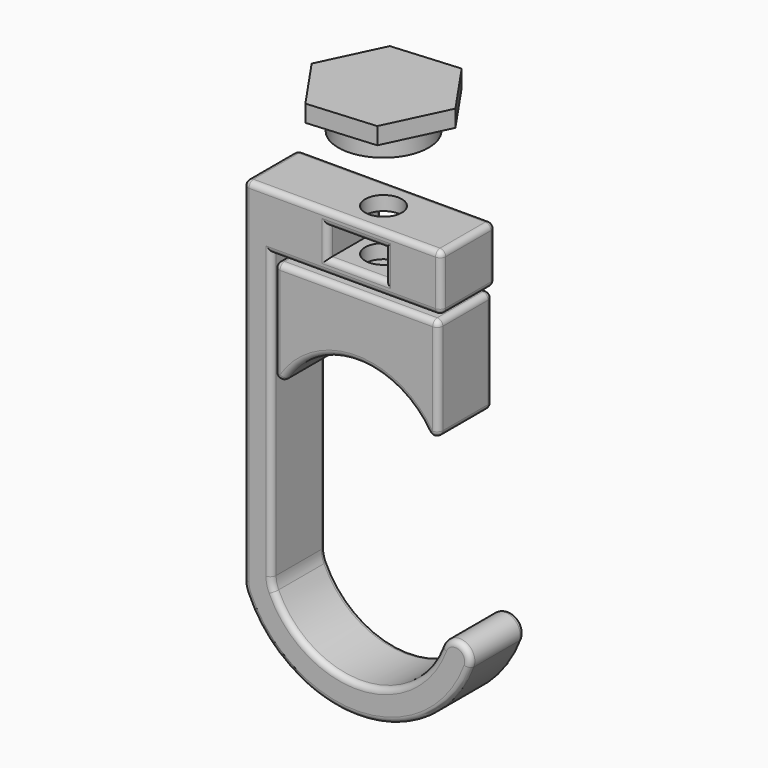
from build123d import *

# Parameters (mm, degrees)
F1_DEPTH  = 6
F3_R      = 3.25
F4_DEPTH  = 15.8
F5_W      = 10.1
F5_H      = 5
F6_DEPTH  = 25
F8_DEPTH  = 5
F10_DEPTH = 12
F12_R     = 1
F12_2_R   = 1


with BuildPart() as f1:
    # F0 (on Front) → F1 (new body, symmetric)
    with BuildSketch(Plane.XZ):
        with BuildLine():
            Line((-15, 0.9851886679), (-15, 51.4083372368))
            Line((-15, 51.4083372368), (15, 51.4083372368))
            Line((15, 51.4083372368), (15, 61.4083372368))
            Line((15, 61.4083372368), (-20, 61.4083372368))
            Line((-20, 61.4083372368), (-20, -0.8958087804))
            ThreePointArc((-20, -0.8958087804), (-19.8968961431, -1.9059613249), (-19.5918367347, -2.8744536202))
            ThreePointArc((-19.5918367347, -2.8744536202), (0.5486358136, -15.7585130867), (20, -1.8559214543))
            ThreePointArc((20, -1.8559214543), (18.4279607271, 1.5720392729), (15, 0))
            ThreePointArc((15, 0), (0.5940911198, -10.4212023249), (-14.5454545455, -1.0978002844))
            ThreePointArc((-14.5454545455, -1.0978002844), (-14.8850421046, -0.0808149139), (-15, 0.9851886679))
        make_face()
    extrude(amount=F1_DEPTH, both=True)


with BuildPart() as f1b:
    # F0 (on Front) → F1, piece 2 (new body, symmetric)
    with BuildSketch(Plane.XZ):
        with BuildLine():
            Line((14.5, 50.4083372368), (-14.5, 50.4083372368))
            Line((-14.5, 50.4083372368), (-14.5, 28.4083372368))
            ThreePointArc((-14.5, 28.4083372368), (0, 39.5677643628), (14.5, 28.4083372368))
            Line((14.5, 28.4083372368), (14.5, 50.4083372368))
        make_face()
    extrude(amount=F1_DEPTH, both=True)


with BuildPart() as f2:
    # F0 (on Front) → F2 (revolve)
    with BuildSketch(Plane.XZ):
        Polygon((12, 80.0677643628), (0, 80.0677643628), (0, 73.0677643628), (8, 73.0677643628), (8, 77.0677643628), (12, 77.0677643628), align=None)
    revolve(axis=Axis((0, 0, 76.5677643628), (0, 0, -1)))

    # F7 (on face) → F8 (cut)
    with BuildSketch(Plane(origin=(0, 0, 73.0677643628), x_dir=(1, 0, 0), z_dir=(0, 0, -1))):
        Polygon((5.05, -2.9156188594), (5.05, 2.9156188594), (0, 5.8312377188), (-5.05, 2.9156188594), (-5.05, -2.9156188594), (0, -5.8312377188), align=None)
    extrude(amount=-F8_DEPTH, mode=Mode.SUBTRACT)


with BuildPart() as f4_tool:
    # F3 (on face) → F4 (new body)
    with BuildSketch(Plane.XY.offset(61.4083372368)):
        Circle(F3_R)
    extrude(amount=-F4_DEPTH)


with BuildPart() as f1_1:
    add(f1.part)

    # F4: cut by f4_tool
    add(f4_tool.part, mode=Mode.SUBTRACT)

    # F5 (on face) → F6 (cut)
    with BuildSketch(Plane.XZ.offset(6)):
        with Locations((0, 56.4083372368)):
            Rectangle(F5_W, F5_H)
    extrude(amount=-F6_DEPTH, mode=Mode.SUBTRACT)

    # F12
    f12_edges = [f1_1.edges().sort_by_distance(p)[0] for p in [
        (-14.885042, -6, -0.080815),
        (0.594091, -6, -10.421202),
        (-15, -6, 26.196763),
        (18.427961, -6, 1.572039),
        (0, -6, 51.408337),
        (0.548636, -6, -15.758513),
        (15, -6, 56.408337),
        (-19.896896, -6, -1.905961),
        (-2.5, -6, 61.408337),
        (-20, -6, 30.256264),
        (0, -6, 58.908337),
        (-5.05, -6, 56.408337),
        (0, -6, 53.908337),
        (5.05, -6, 56.408337),
        (-14.885042, 6, -0.080815),
        (0.594091, 6, -10.421202),
        (-15, 6, 26.196763),
        (18.427961, 6, 1.572039),
        (0, 6, 51.408337),
        (0.548636, 6, -15.758513),
        (15, 6, 56.408337),
        (-19.896896, 6, -1.905961),
        (-2.5, 6, 61.408337),
        (-20, 6, 30.256264),
        (0, 6, 58.908337),
        (-5.05, 6, 56.408337),
        (0, 6, 53.908337),
        (5.05, 6, 56.408337),
        (15, 0, 51.408337),
        (15, 0, 61.408337),
        (-20, 0, 61.408337),
        (-20, 0, -0.895809),
    ]]
    fillet(f12_edges, radius=F12_R)


with BuildPart() as f1b_1:
    add(f1b.part)

    # F4: cut by f4_tool
    add(f4_tool.part, mode=Mode.SUBTRACT)

    # F12#2
    f12_2_edges = [f1b_1.edges().sort_by_distance(p)[0] for p in [
        (14.5, -6, 39.408337),
        (0, -6, 50.408337),
        (-14.5, -6, 39.408337),
        (0, -6, 39.567764),
        (14.5, 6, 39.408337),
        (0, 6, 50.408337),
        (-14.5, 6, 39.408337),
        (0, 6, 39.567764),
        (14.5, 0, 50.408337),
        (14.5, 0, 28.408337),
        (-14.5, 0, 50.408337),
        (-14.5, 0, 28.408337),
    ]]
    fillet(f12_2_edges, radius=F12_2_R)


with BuildPart() as f10:
    # F9 (on face) → F10 (new body)
    with BuildSketch(Plane.XY.offset(80.0677643628)):
        Polygon((11.9626500532, 0.9460463543), (5.1620248506, 10.8329820198), (-6.8006252026, 9.8869356655), (-11.9626500532, -0.9460463543), (-5.1620248506, -10.8329820198), (6.8006252026, -9.8869356655), align=None)
    extrude(amount=-F10_DEPTH)


with BuildPart() as f2_1:
    add(f2.part)

    # F11: intersect F10
    add(f10.part, mode=Mode.INTERSECT)


solid = Compound([f1_1.part, f1b_1.part, f2_1.part])
